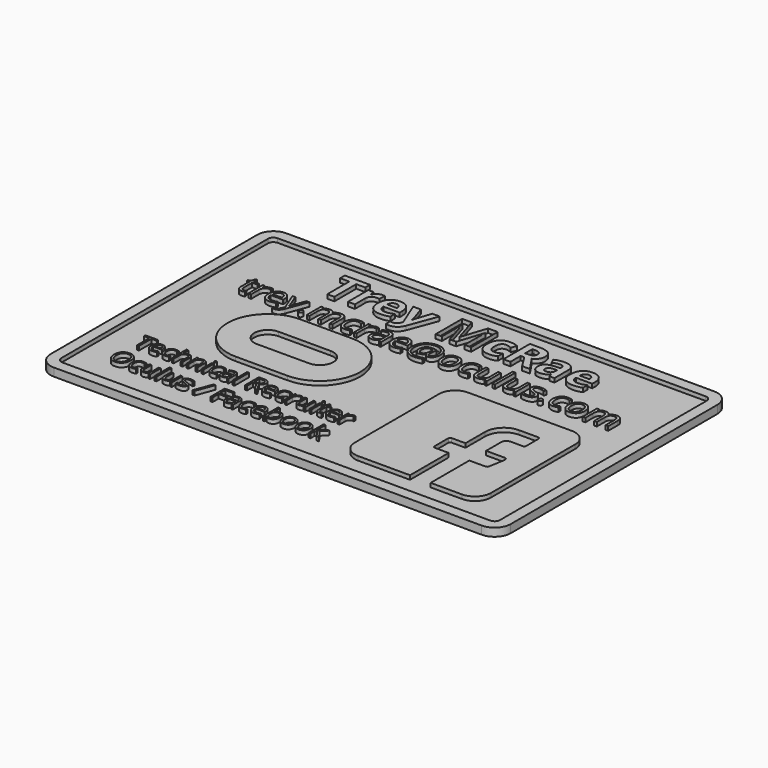
from build123d import *

# Parameters (mm, degrees)
F7_DEPTH     = 0.75
F6_TEXT_SIZE = 4.6465196479
F4_TEXT_SIZE = 6.2384247977
F3_TEXT_SIZE = 8.6407085381
F5_TEXT_SIZE = 4.4846977209
F8_DEPTH     = 1.5


# Not quite as in the source:
# - Text() gives the source's letters only with a copy of the font that has no kerning and outlines rounded to 1/6400 em; it was checked with that copy


with BuildPart() as f7:
    # F0 (on Top) → F7 (new body)
    with BuildSketch(Plane.XY):
        with BuildLine():
            Line((39.75, 23.1077305627), (-39.75, 23.1077305627))
            ThreePointArc((-39.75, 23.1077305627), (-40.4571067812, 22.8148373439), (-40.75, 22.1077305627))
            Line((-40.75, 22.1077305627), (-40.75, -25.8922694373))
            ThreePointArc((-40.75, -25.8922694373), (-40.4571067812, -26.5993762185), (-39.75, -26.8922694373))
            Line((-39.75, -26.8922694373), (39.75, -26.8922694373))
            ThreePointArc((39.75, -26.8922694373), (40.4571067812, -26.5993762185), (40.75, -25.8922694373))
            Line((40.75, -25.8922694373), (40.75, 22.1077305627))
            ThreePointArc((40.75, 22.1077305627), (40.4571067812, 22.8148373439), (39.75, 23.1077305627))
        make_face()
    extrude(amount=F7_DEPTH)

    # F0 (on Top) + F1 (on Top) + F2 (on Top) + F6 (on Top) + F4 (on Top) + F3 (on Top) + F5 (on Top) → F8 (join)
    with BuildSketch(Plane.XY):
        with BuildLine():
            Line((39.75, 25.1077305627), (-39.75, 25.1077305627))
            ThreePointArc((-39.75, 25.1077305627), (-41.8713203436, 24.2290509062), (-42.75, 22.1077305627))
            Line((-42.75, 22.1077305627), (-42.75, -25.8922694373))
            ThreePointArc((-42.75, -25.8922694373), (-41.8713203436, -28.0135897809), (-39.75, -28.8922694373))
            Line((-39.75, -28.8922694373), (39.75, -28.8922694373))
            ThreePointArc((39.75, -28.8922694373), (41.8713203436, -28.0135897809), (42.75, -25.8922694373))
            Line((42.75, -25.8922694373), (42.75, 22.1077305627))
            ThreePointArc((42.75, 22.1077305627), (41.8713203436, 24.2290509062), (39.75, 25.1077305627))
        make_face()
        with BuildLine():
            ThreePointArc((-40.75, 22.1077305627), (-40.4571067812, 22.8148373439), (-39.75, 23.1077305627))
            Line((-39.75, 23.1077305627), (39.75, 23.1077305627))
            ThreePointArc((39.75, 23.1077305627), (40.4571067812, 22.8148373439), (40.75, 22.1077305627))
            Line((40.75, 22.1077305627), (40.75, -25.8922694373))
            ThreePointArc((40.75, -25.8922694373), (40.4571067812, -26.5993762185), (39.75, -26.8922694373))
            Line((39.75, -26.8922694373), (-39.75, -26.8922694373))
            ThreePointArc((-39.75, -26.8922694373), (-40.4571067812, -26.5993762185), (-40.75, -25.8922694373))
            Line((-40.75, -25.8922694373), (-40.75, 22.1077305627))
        make_face(mode=Mode.SUBTRACT)
    with BuildSketch(Plane.XY):
        with BuildLine():
            Line((31.4093656167, 2.5085634552), (12.0937996283, 2.5085634552))
            ThreePointArc((12.0937996283, 2.5085634552), (9.9724792848, 1.6298837988), (9.0937996283, -0.4914365448))
            Line((9.0937996283, -0.4914365448), (9.0937996283, -20.0372585356))
            ThreePointArc((9.0937996283, -20.0372585356), (9.9724792848, -22.1585788792), (12.0937996283, -23.0372585356))
            Line((12.0937996283, -23.0372585356), (21.7515826225, -23.0372585356))
            Line((21.7515826225, -23.0372585356), (21.7515826225, -14.0581438318))
            Line((21.7515826225, -14.0581438318), (19.1341364264, -14.0581438318))
            ThreePointArc((19.1341364264, -14.0581438318), (18.9220043921, -13.9702758661), (18.8341364264, -13.7581438318))
            Line((18.8341364264, -13.7581438318), (18.8341364264, -10.45761399))
            ThreePointArc((18.8341364264, -10.45761399), (18.9220043921, -10.2454819557), (19.1341364264, -10.15761399))
            Line((19.1341364264, -10.15761399), (21.7515826225, -10.15761399))
            Line((21.7515826225, -10.15761399), (21.7515826225, -5.6088223439))
            ThreePointArc((21.7515826225, -5.6088223439), (22.7767088884, -3.1339486097), (25.2515826225, -2.1088223439))
            Line((25.2515826225, -2.1088223439), (28.8716940053, -2.1088223439))
            ThreePointArc((28.8716940053, -2.1088223439), (29.0838260397, -2.1966903095), (29.1716940053, -2.4088223439))
            Line((29.1716940053, -2.4088223439), (29.1716940053, -5.3830801574))
            ThreePointArc((29.1716940053, -5.3830801574), (29.0838260397, -5.5952121918), (28.8716940053, -5.6830801574))
            Line((28.8716940053, -5.6830801574), (26.584375026, -5.6830801574))
            ThreePointArc((26.584375026, -5.6830801574), (25.8772682448, -5.9759733762), (25.584375026, -6.6830801574))
            Line((25.584375026, -6.6830801574), (25.584375026, -10.15761399))
            Line((25.584375026, -10.15761399), (28.9974417876, -10.15761399))
            ThreePointArc((28.9974417876, -10.15761399), (29.3797737985, -10.3353994134), (29.4902135757, -10.7423250564))
            Line((29.4902135757, -10.7423250564), (28.9773130896, -13.7259126849))
            ThreePointArc((28.9773130896, -13.7259126849), (28.8408673204, -13.9640094406), (28.5830956591, -14.0581438318))
            Line((28.5830956591, -14.0581438318), (25.584375026, -14.0581438318))
            Line((25.584375026, -14.0581438318), (25.584375026, -23.0372585356))
            Line((25.584375026, -23.0372585356), (31.4093656167, -23.0372585356))
            ThreePointArc((31.4093656167, -23.0372585356), (33.5306859603, -22.1585788792), (34.4093656167, -20.0372585356))
            Line((34.4093656167, -20.0372585356), (34.4093656167, -0.4914365448))
            ThreePointArc((34.4093656167, -0.4914365448), (33.5306859603, 1.6298837988), (31.4093656167, 2.5085634552))
        make_face()
    with BuildSketch(Plane.XY):
        with BuildLine():
            ThreePointArc((-21.3126111776, 5.2594595402), (-28.8126111776, -2.2405404598), (-21.3126111776, -9.7405404598))
            Line((-21.3126111776, -9.7405404598), (-11.6418842226, -9.7405404598))
            ThreePointArc((-11.6418842226, -9.7405404598), (-4.1418842226, -2.2405404598), (-11.6418842226, 5.2594595402))
            Line((-11.6418842226, 5.2594595402), (-21.3126111776, 5.2594595402))
        make_face()
        with BuildLine():
            Line((-11.6303116083, -4.7405404598), (-21.3115867227, -4.7405404598))
            ThreePointArc((-21.3115867227, -4.7405404598), (-23.8115867227, -2.2405404598), (-21.3115867227, 0.2594595402))
            Line((-21.3115867227, 0.2594595402), (-11.6303116083, 0.2594595402))
            ThreePointArc((-11.6303116083, 0.2594595402), (-9.1303116083, -2.2405404598), (-11.6303116083, -4.7405404598))
        make_face(mode=Mode.SUBTRACT)
    with BuildSketch(Plane.XY):
        with Locations((-35.75, -21.8922694373)):
            Text('Oculus / Facebook', F6_TEXT_SIZE, font='Open Sans', text_align=(TextAlign.LEFT, TextAlign.BOTTOM))
    with BuildSketch(Plane.XY):
        with Locations((-35, 6.938282866)):
            Text('trey.mcrae@oculus.com', F4_TEXT_SIZE, font='Open Sans', text_align=(TextAlign.LEFT, TextAlign.BOTTOM))
    with BuildSketch(Plane.XY):
        with Locations((-25, 13.8864204153)):
            Text('Trey McRae', F3_TEXT_SIZE, font='Open Sans', font_style=FontStyle.BOLD, text_align=(TextAlign.LEFT, TextAlign.BOTTOM))
    with BuildSketch(Plane.XY):
        with Locations((-35.75, -15.8922694373)):
            Text('Technical Recruiter', F5_TEXT_SIZE, font='Open Sans', text_align=(TextAlign.LEFT, TextAlign.BOTTOM))
    extrude(amount=F8_DEPTH)


solid = f7.part
